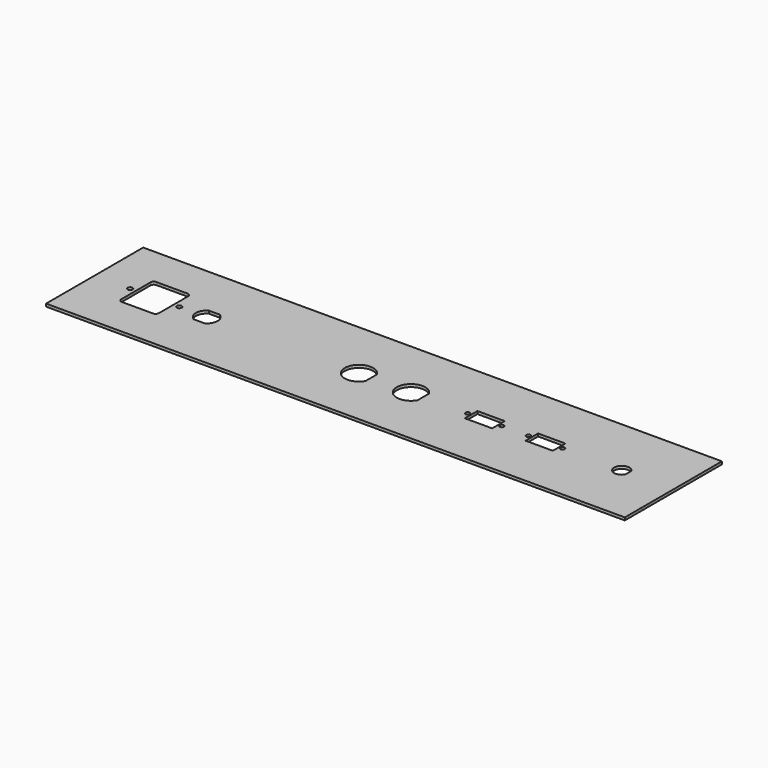
from build123d import *

# Parameters (mm, degrees)
F0_W     = 423.8752
F0_H     = 88.9
F1_DEPTH = 2
F2_R     = 1.8
F2_W     = 20.0025
F2_H     = 11.50112
F2_R_2   = 1.6
F3_DEPTH = 25.4


# Not quite as in the source:
# - a feature names something its author has since deleted; it is built from what else it names


with BuildPart() as f1:
    # F0 (on Top) → F1 (new body)
    with BuildSketch(Plane.XY):
        with Locations((20.2464647591, -83.8722900312)):
            Rectangle(F0_W, F0_H)
    extrude(amount=F1_DEPTH)

    # F2 (on face) → F3 (cut)
    with BuildSketch(Plane.XY.offset(2)):
        with Locations((-165.6916952409, -83.8722900312)):
            Circle(F2_R)
        with BuildLine():
            Line((-159.0907152409, -99.6722900312), (-136.2907152409, -99.6722900312))
            ThreePointArc((-136.2907152409, -99.6722900312), (-134.593658966, -98.9693463061), (-133.8907152409, -97.2722900312))
            Line((-133.8907152409, -97.2722900312), (-133.8907152409, -70.4722900312))
            ThreePointArc((-133.8907152409, -70.4722900312), (-134.593658966, -68.7752337564), (-136.2907152409, -68.0722900312))
            Line((-136.2907152409, -68.0722900312), (-159.0907152409, -68.0722900312))
            ThreePointArc((-159.0907152409, -68.0722900312), (-160.7877715157, -68.7752337564), (-161.4907152409, -70.4722900312))
            Line((-161.4907152409, -70.4722900312), (-161.4907152409, -97.2722900312))
            ThreePointArc((-161.4907152409, -97.2722900312), (-160.7877715157, -98.9693463061), (-159.0907152409, -99.6722900312))
        make_face()
        with Locations((-129.6922752409, -83.8722900312)):
            Circle(F2_R)
        with BuildLine():
            ThreePointArc((-105.5771334553, -90.7937900312), (-102.6578706275, -87.8662437824), (-101.5897152409, -83.8722900312))
            ThreePointArc((-101.5897152409, -83.8722900312), (-102.6578706275, -79.87833628), (-105.5771334553, -76.9507900312))
            Line((-105.5771334553, -76.9507900312), (-113.6042970265, -76.9507900312))
            ThreePointArc((-113.6042970265, -76.9507900312), (-117.5917152409, -83.8722900312), (-113.6042970265, -90.7937900312))
            Line((-113.6042970265, -90.7937900312), (-105.5771334553, -90.7937900312))
        make_face()
        with BuildLine():
            Line((10.8975047591, -89.0838157195), (10.8975047591, -78.6607643429))
            ThreePointArc((10.8975047591, -78.6607643429), (-8.5024952409, -83.8722900312), (10.8975047591, -89.0838157195))
        make_face()
        with BuildLine():
            Line((48.9975047591, -89.0838157195), (48.9975047591, -78.6607643429))
            ThreePointArc((48.9975047591, -78.6607643429), (29.5975047591, -83.8722900312), (48.9975047591, -89.0838157195))
        make_face()
        with BuildLine():
            Line((199.2388647591, -86.5704375439), (199.2388647591, -81.1741425186))
            ThreePointArc((199.2388647591, -81.1741425186), (188.8388647591, -83.8722900312), (199.2388647591, -86.5704375439))
        make_face()
        with Locations((94.0588647591, -83.8722900312)):
            Rectangle(F2_W, F2_H)
        with Locations((138.5088647591, -83.8722900312)):
            Rectangle(F2_W, F2_H)
        with Locations((106.5582047591, -83.8722900312)):
            Circle(F2_R_2)
        with Locations((81.5595247591, -83.8722900312)):
            Circle(F2_R_2)
        with Locations((126.0095247591, -83.8722900312)):
            Circle(F2_R_2)
        with Locations((151.0082047591, -83.8722900312)):
            Circle(F2_R_2)
    extrude(amount=-F3_DEPTH, mode=Mode.SUBTRACT)


solid = f1.part
